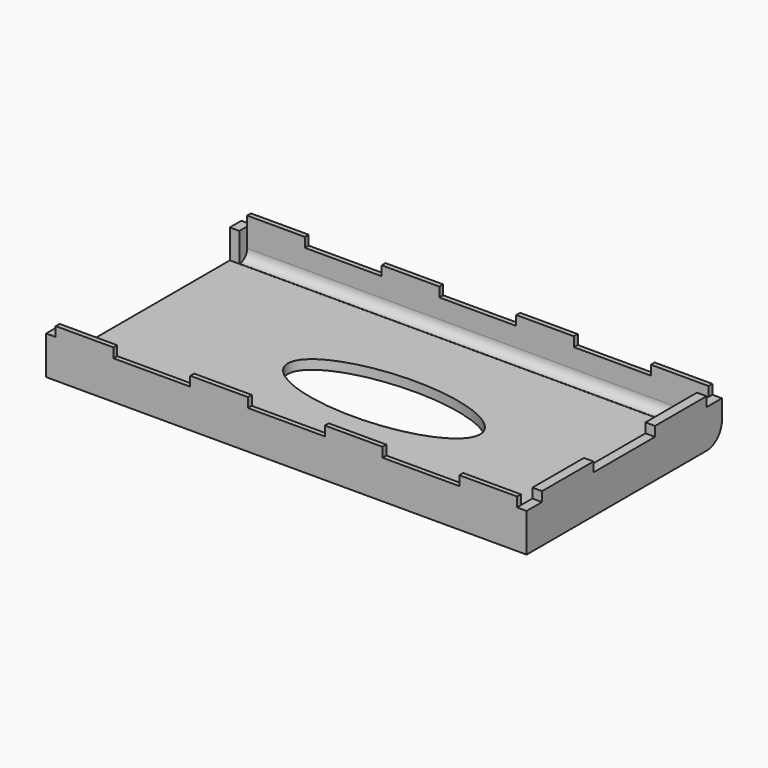
from build123d import *

# Parameters (mm, degrees)
F0_W     = 158.75
F0_H     = 80.645
F1_DEPTH = 15.875
F2_W     = 71.12
F2_H     = 9.652
F3_DEPTH = 155.575
F5_DEPTH = 12.7
F6_W     = 3.175
F6_H     = 40.3225
F6_W_2   = 25.4
F6_H_2   = 1.5875
F6_H_3   = 6.35
F6_H_4   = 25.4
F7_DEPTH = 3.175
F9_DEPTH = 25.4
F10_R    = 3.17499
F11_R    = 6.35


# Not quite as in the source:
# - a fillet or chamfer is up to 0.001 mm smaller than in the source, because OpenCascade refuses the exact size


with BuildPart() as f1:
    # F0 (on Top) → F1 (new body)
    with BuildSketch(Plane.XY):
        Rectangle(F0_W, F0_H)
    extrude(amount=F1_DEPTH)

    # F2 (on face) → F3 (cut)
    with BuildSketch(Plane(origin=(-79.375, 0, 0), x_dir=(0, -1, 0), z_dir=(-1, 0, 0))):
        with Locations((0, 7.9375)):
            Rectangle(F2_W, F2_H)
    extrude(amount=-F3_DEPTH, mode=Mode.SUBTRACT)

    # F4 (on face) → F5 (cut)
    with BuildSketch(Plane.XY.offset(15.875)):
        Polygon((76.2, 38.735), (-76.2, 38.735), (-76.2, 0), (-76.2, -38.735), (76.2, -38.735), align=None)
    extrude(amount=-F5_DEPTH, mode=Mode.SUBTRACT)

    # F6 (on face) → F7 (cut)
    with BuildSketch(Plane.XY.offset(15.875)):
        with Locations((-77.7875, -20.16125)):
            Rectangle(F6_W, F6_H)
        with Locations((-77.7875, 20.16125)):
            Rectangle(F6_W, F6_H)
        with Locations((-44.45, -39.52875)):
            Rectangle(F6_W_2, F6_H_2)
        with Locations((0, -39.52875)):
            Rectangle(F6_W_2, F6_H_2)
        with Locations((44.45, -39.52875)):
            Rectangle(F6_W_2, F6_H_2)
        with Locations((-44.45, 39.52875)):
            Rectangle(F6_W_2, F6_H_2)
        with Locations((0, 39.52875)):
            Rectangle(F6_W_2, F6_H_2)
        with Locations((44.45, 39.52875)):
            Rectangle(F6_W_2, F6_H_2)
        with Locations((77.7875, 37.1475)):
            Rectangle(F6_W, F6_H_3)
        with Locations((77.7875, -37.1475)):
            Rectangle(F6_W, F6_H_3)
        with Locations((77.7875, 0)):
            Rectangle(F6_W, F6_H_4)
    extrude(amount=-F7_DEPTH, mode=Mode.SUBTRACT)

    # F8 (on face) → F9 (cut)
    with BuildSketch(Plane.XY.offset(3.1115)):
        with BuildLine():
            add(Edge.make_bspline(
                [(-31.75, 0), (-31.75, -21.9970452561), (15.875, -10.9985226281), (63.5, 0), (15.875, 10.9985226281), (-31.75, 21.9970452561), (-31.75, 0)],
                knots=[0, 0, 0, 2.0943951024, 2.0943951024, 4.1887902048, 4.1887902048, 6.2831853072, 6.2831853072, 6.2831853072], degree=2, weights=[1, 0.5, 1, 0.5, 1, 0.5, 1]))
        make_face()
    extrude(amount=-F9_DEPTH, mode=Mode.SUBTRACT)

    # F10 (radius 3.175 in the source; OpenCascade refuses exactly that, so slightly less here)
    f10_edges = [f1.edges().sort_by_distance(p)[0] for p in [
        (0, 38.735, 3.175),
    ]]
    fillet(f10_edges, radius=F10_R)

    # F11
    f11_edges = [f1.edges().sort_by_distance(p)[0] for p in [
        (0, 40.3225, 0),
    ]]
    fillet(f11_edges, radius=F11_R)


solid = f1.part
